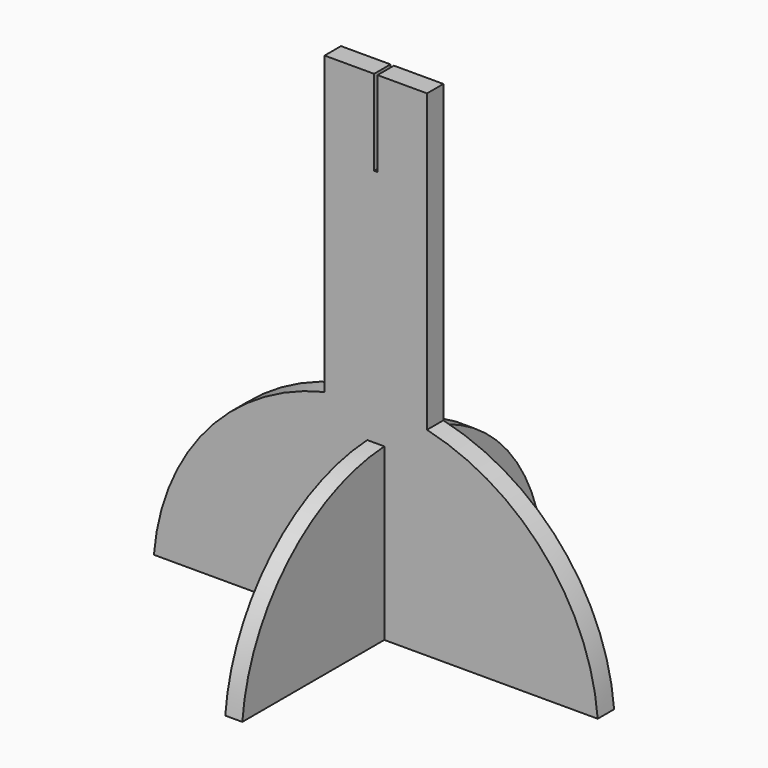
from build123d import *

# Parameters (mm, degrees)
F0_W     = 7.25
F0_H     = 12.5
F1_DEPTH = 3
F3_DEPTH = 2.5


with BuildPart() as f1:
    # F0 (on Front) → F1 (new body)
    with BuildSketch(Plane.XZ):
        with BuildLine():
            ThreePointArc((-7.5, 29.125656592), (-24.7401691178, 18.6315512644), (-32.5, 0))
            Line((-32.5, 0), (-7.5, 0))
            Line((-7.5, 0), (-7.5, 29.125656592))
        make_face()
        with BuildLine():
            Line((-7.5, 29.125656592), (-7.5, 0))
            Line((-7.5, 0), (-1.25, 0))
            Line((-1.25, 0), (-1.25, 17.5))
            Line((-1.25, 17.5), (0, 17.5))
            Line((0, 17.5), (0, 30))
            ThreePointArc((0, 30), (-3.7753965485, 29.7806764691), (-7.5, 29.125656592))
        make_face()
        with BuildLine():
            Line((-7.5, 60), (-7.5, 29.125656592))
            ThreePointArc((-7.5, 29.125656592), (-3.7753965485, 29.7806764691), (0, 30))
            ThreePointArc((0, 30), (3.7753965485, 29.7806764691), (7.5, 29.125656592))
            Line((7.5, 29.125656592), (7.5, 60))
            Line((7.5, 60), (0.25, 60))
            Line((0.25, 60), (-0.25, 60))
            Line((-0.25, 60), (-7.5, 60))
        make_face()
        with BuildLine():
            ThreePointArc((7.5, 29.125656592), (3.7753965485, 29.7806764691), (0, 30))
            Line((0, 30), (0, 17.5))
            Line((0, 17.5), (1.25, 17.5))
            Line((1.25, 17.5), (1.25, 0))
            Line((1.25, 0), (7.5, 0))
            Line((7.5, 0), (7.5, 29.125656592))
        make_face()
        with Locations((-3.875, 66.25)):
            Rectangle(F0_W, F0_H)
        with BuildLine():
            ThreePointArc((32.5, 0), (24.7401691178, 18.6315512644), (7.5, 29.125656592))
            Line((7.5, 29.125656592), (7.5, 0))
            Line((7.5, 0), (32.5, 0))
        make_face()
        with Locations((3.875, 66.25)):
            Rectangle(F0_W, F0_H)
    extrude(amount=F1_DEPTH)


with BuildPart() as f3:
    # F2 (on face) → F3 (new body)
    with BuildSketch(Plane.YZ.offset(-1.25)):
        Polygon((-3, 17.5), (-3, 0), (-1.5, 0), (0, 0), (0, 17.5), align=None)
        with BuildLine():
            Line((-29, 0), (-3, 0))
            Line((-3, 0), (-3, 17.5))
            Line((-3, 17.5), (-3, 24.9592459567))
            ThreePointArc((-3, 24.9592459567), (-20.6308909798, 17.3036134821), (-29, 0))
        make_face()
        with BuildLine():
            Line((0, 24.9592459567), (0, 17.5))
            Line((0, 17.5), (0, 0))
            Line((0, 0), (26, 0))
            ThreePointArc((26, 0), (17.6308909798, 17.3036134821), (0, 24.9592459567))
        make_face()
    extrude(amount=F3_DEPTH)


solid = Compound([f1.part, f3.part])
